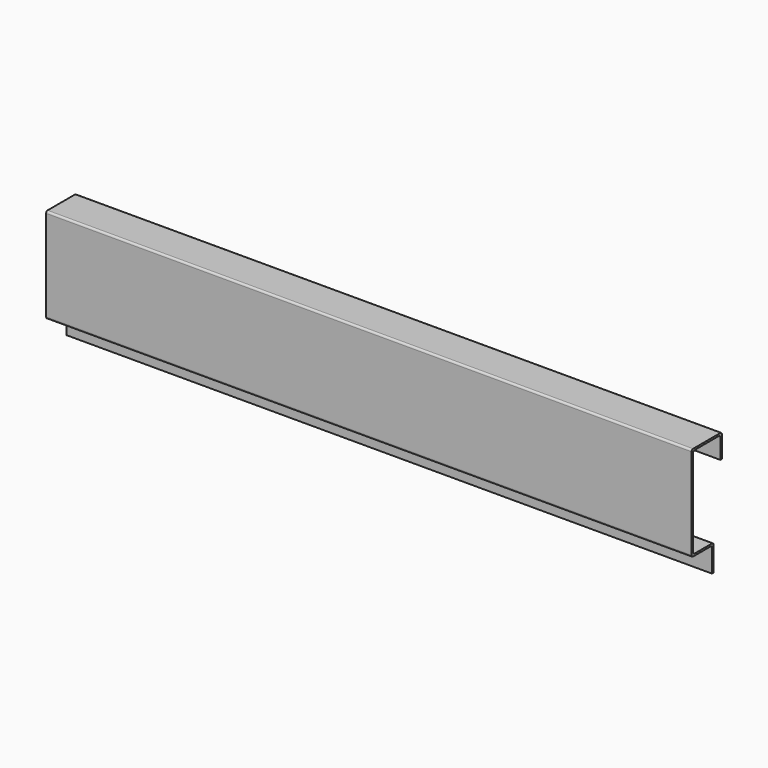
from build123d import *

# Parameters (mm, degrees)
F1_DEPTH = 680
F3_D     = 5
F4_R     = 2


# Not quite as in the source:
# - a feature names something its author has since deleted; it is built from what else it names


with BuildPart() as f1:
    # F0 (on Right) → F1 (new body)
    with BuildSketch(Plane.YZ):
        Polygon((-18.8378913403, 177.8021101952), (-18.8378913403, 154.8021101952), (-16.8378913403, 154.8021101952), (-16.8378913403, 179.8021101952), (-56.8378913403, 179.8021101952), (-56.8378913403, 79.8021101952), (-29.8378913403, 79.8021101952), (-29.8378913403, 53.8021101952), (-27.8378913403, 53.8021101952), (-27.8378913403, 81.8021101952), (-54.8378913403, 81.8021101952), (-54.8378913403, 177.8021101952), align=None)
    extrude(amount=F1_DEPTH)

    # F3 (through all)
    with Locations(Plane.XZ.offset(29.8378913403)):
        with Locations((580, 66.8021101952), (100, 66.8021101952)):
            Hole(F3_D / 2)

    # F4
    f4_edges = [f1.edges().sort_by_distance(p)[0] for p in [
        (340, -56.837891, 179.80211),
        (340, -16.837891, 179.80211),
        (340, -56.837891, 79.80211),
        (340, -27.837891, 81.80211),
        (340, -54.837891, 81.80211),
        (340, -29.837891, 79.80211),
        (340, -18.837891, 177.80211),
        (340, -54.837891, 177.80211),
    ]]
    fillet(f4_edges, radius=F4_R)


solid = f1.part
